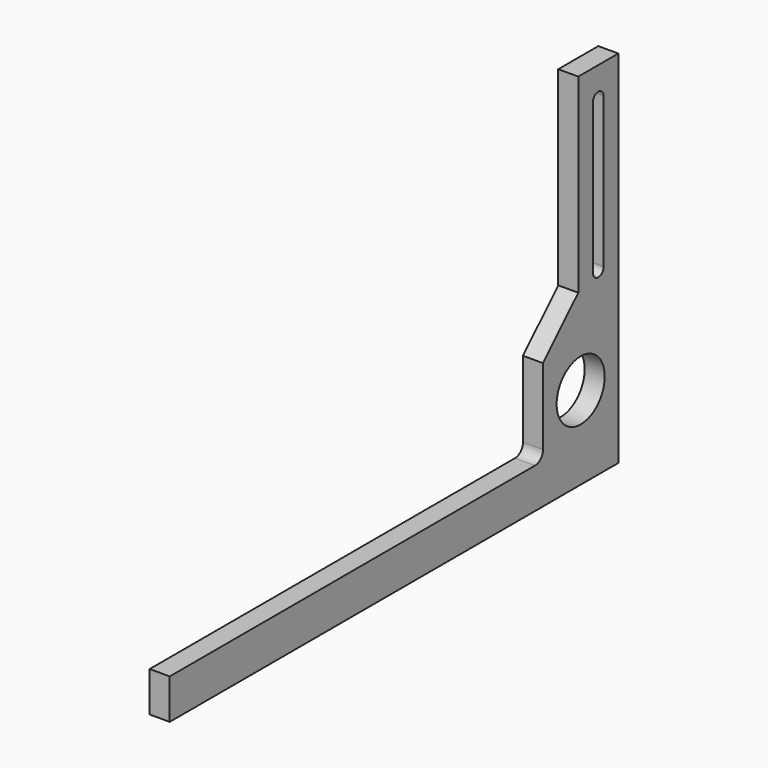
from build123d import *

# Parameters (mm, degrees)
F0_R     = 19.05
F1_DEPTH = 12.7
F3_DEPTH = 12.701


# Not quite as in the source:
# - a feature names something its author has since deleted; it is built from what else it names


with BuildPart() as f1:
    # F0 (on Right) → F1 (new body)
    with BuildSketch(Plane.YZ):
        with BuildLine():
            Line((111.75, 25.4), (-177.8, 25.4))
            Line((-177.8, 25.4), (-177.8, 0))
            Line((-177.8, 0), (146.05, 0))
            Line((146.05, 0), (177.8, 0))
            Line((177.8, 0), (177.8, 25.4))
            Line((177.8, 25.4), (177.8, 228.6))
            Line((177.8, 228.6), (146.05, 228.6))
            Line((146.05, 228.6), (146.05, 107.95))
            Line((146.05, 107.95), (118.1, 80))
            Line((118.1, 80), (118.1, 31.75))
            ThreePointArc((118.1, 31.75), (116.2401280605, 27.2598719395), (111.75, 25.4))
        make_face()
        with Locations((147.9499962, 52.7)):
            Circle(F0_R, mode=Mode.SUBTRACT)
    extrude(amount=F1_DEPTH)

    # F2 (on face) → F3 (cut, through all)
    with BuildSketch(Plane.YZ.offset(12.7)):
        with BuildLine():
            ThreePointArc((166.1414, 209.55), (161.925, 213.7664), (157.7086, 209.55))
            Line((157.7086, 209.55), (157.7086, 114.3))
            ThreePointArc((157.7086, 114.3), (161.925, 110.0836), (166.1414, 114.3))
            Line((166.1414, 114.3), (166.1414, 209.55))
        make_face()
    extrude(amount=-F3_DEPTH, mode=Mode.SUBTRACT)


solid = f1.part
